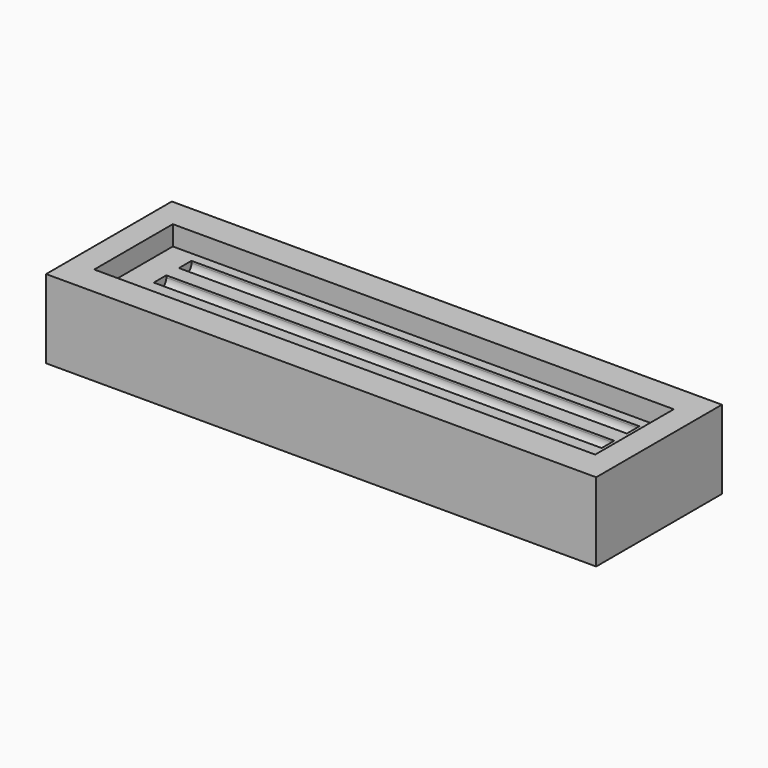
from build123d import *

# Parameters (mm, degrees)
F0_W     = 35.56
F0_H     = 10.16
F1_DEPTH = 5.08
F2_W     = 32.385
F2_H     = 6.35
F3_DEPTH = 1.27
F4_W     = 28.956
F4_H     = 1.016
F5_DEPTH = 0.635
F6_R     = 0.50799


# Not quite as in the source:
# - a fillet or chamfer is up to 0.001 mm smaller than in the source, because OpenCascade refuses the exact size


with BuildPart() as f1:
    # F0 (on Top) → F1 (new body)
    with BuildSketch(Plane.XY):
        Rectangle(F0_W, F0_H)
    extrude(amount=F1_DEPTH)

    # F2 (on face) → F3 (cut)
    with BuildSketch(Plane.XY.offset(5.08)):
        Rectangle(F2_W, F2_H)
    extrude(amount=-F3_DEPTH, mode=Mode.SUBTRACT)

    # F4 (on face) → F5 (cut)
    with BuildSketch(Plane.XY.offset(3.81)):
        Rectangle(F4_W, F4_H)
        with Locations((0, 2.032)):
            Rectangle(F4_W, F4_H)
        with Locations((0, -1.778)):
            Rectangle(F4_W, F4_H)
    extrude(amount=-F5_DEPTH, mode=Mode.SUBTRACT)

    # F6 (radius 0.508 in the source; OpenCascade refuses exactly that, so slightly less here)
    f6_edges = [f1.edges().sort_by_distance(p)[0] for p in [
        (0, 0.508, 3.175),
        (0, -0.508, 3.175),
        (0, 2.54, 3.175),
        (0, -1.27, 3.175),
        (0, 1.524, 3.175),
        (0, -2.286, 3.175),
    ]]
    fillet(f6_edges, radius=F6_R)


solid = f1.part
